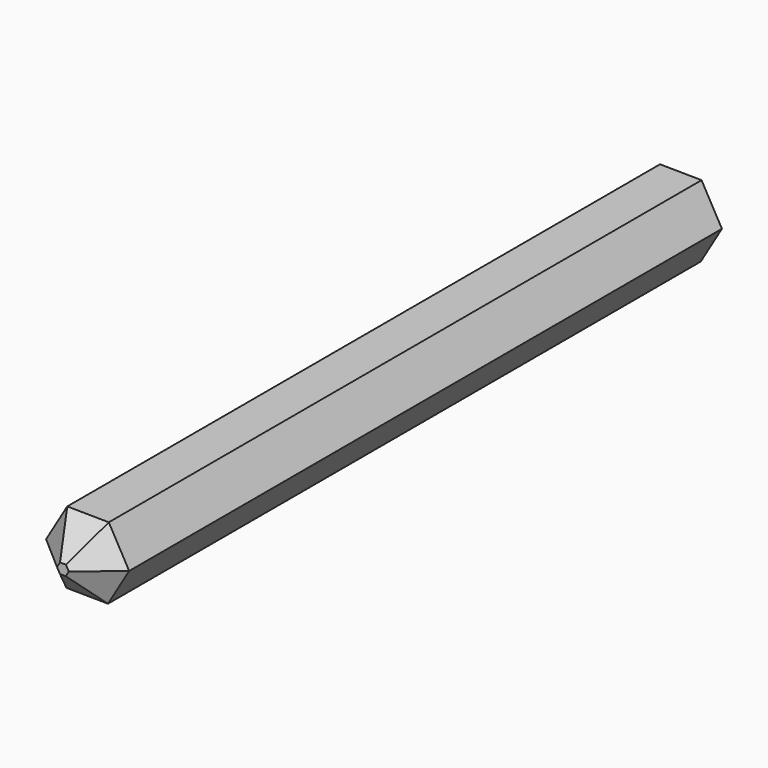
from build123d import *

# Parameters (mm, degrees)
F2_DEPTH = 127
F4_SIZE  = 5.08


# Not quite as in the source:
# - the program builds the solid bodies; features that only make, move or delete a surface that nothing else refers to are left out


with BuildPart() as f2:
    # F1 (on Front) → F2 (new body)
    with BuildSketch(Plane.XZ):
        Polygon((6.8357169452, -0.0776342775), (3.4850917291, 5.8810873888), (-3.3506252161, 5.9587216663), (-6.8357169452, 0.0776342775), (-3.4850917291, -5.8810873888), (3.3506252161, -5.9587216663), align=None)
    extrude(amount=F2_DEPTH)

    # F4
    f4_edges = [f2.edges().sort_by_distance(p)[0] for p in [
        (5.160404, -127, 2.901727),
        (0.067233, -127, 5.919905),
        (-5.093171, -127, 3.018178),
        (-5.160404, -127, -2.901727),
        (-0.067233, -127, -5.919905),
        (5.093171, -127, -3.018178),
    ]]
    chamfer(f4_edges, length=F4_SIZE)


solid = f2.part
